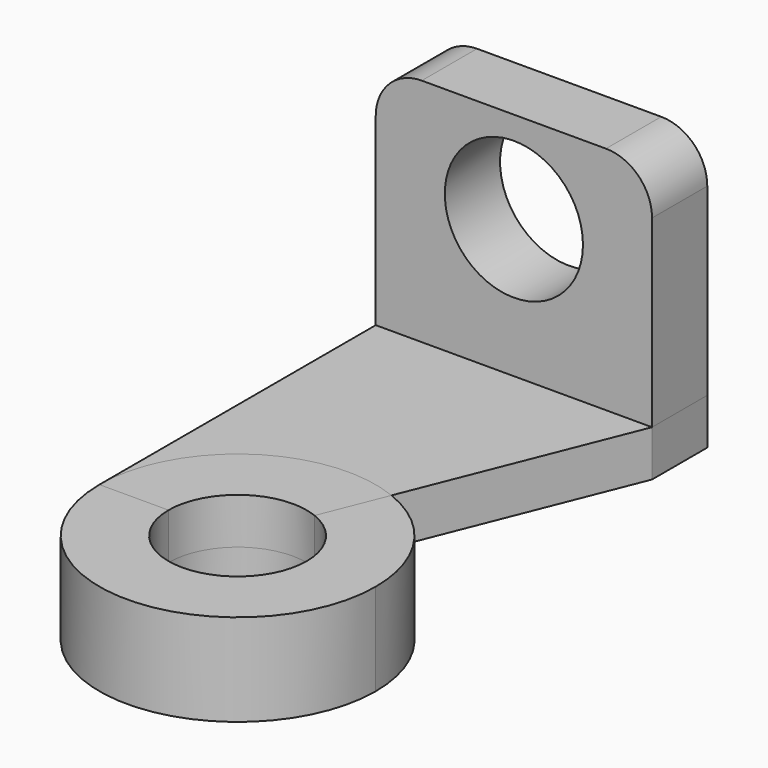
from build123d import *
from build123d import SkipClean  # not in build123d's __all__

# Parameters (mm, degrees)
F1_DEPTH      = 15
F2_R          = 15
F3_DEPTH      = 25
F3_DEPTH_BACK = 25
F6_DEPTH      = 10
F7_DEPTH      = 15
F9_DEPTH      = 10
F10_DEPTH     = 20
F11_DEPTH     = 20


with BuildPart() as f1:
    # F0 (on Front) → F1 (new body)
    with BuildSketch(Plane.XZ):
        with BuildLine():
            ThreePointArc((30, 15), (27.0710678119, 22.0710678119), (20, 25))
            Line((20, 25), (-20, 25))
            ThreePointArc((-20, 25), (-27.0710678119, 22.0710678119), (-30, 15))
            Line((-30, 15), (-30, -25))
            Line((-30, -25), (30, -25))
            Line((30, -25), (30, 15))
        make_face()
    extrude(amount=F1_DEPTH)


with BuildPart() as f3:
    # F2 (on face) → F3 (new body, two sides)
    with BuildSketch(Plane.XZ.offset(15)) as f3_sk:
        with Locations((0, 5)):
            Circle(F2_R)
    extrude(amount=-F3_DEPTH)
    extrude(f3_sk.sketch, amount=F3_DEPTH_BACK)


with BuildPart() as f1_1:
    add(f1.part, clean=False)

    # F4: cut F3
    add(f3.part, mode=Mode.SUBTRACT)



with BuildPart() as f6:
    # F5 (on face) → F6 (new body)
    with BuildSketch(Plane(origin=(0, 0, -25), x_dir=(1, 0, 0), z_dir=(0, 0, -1))):
        Polygon((-30, 90), (-30, 15), (30, 15), (0, 90), align=None)
    extrude(amount=F6_DEPTH)


with BuildPart() as f7:
    # F7 (new): a face of the model
    f7_faces = [f6.part.faces().sort_by_distance(p)[0] for p in [
        (0, -15, -30),
    ]]
    extrude(f7_faces, amount=F7_DEPTH)


with BuildPart() as f6_1:
    add(f6.part, clean=False)

    # F8 (on face) → F9 (cut)
    with BuildSketch(Plane.XY.offset(-25)):
        with BuildLine():
            ThreePointArc((5.5708601453, -76.0728496367), (-8.4094321396, -77.578991543), (-15, -90))
            Line((-15, -90), (0, -90))
            Line((0, -90), (5.5708601453, -76.0728496367))
        make_face()
    extrude(amount=-F9_DEPTH, mode=Mode.SUBTRACT)


with BuildPart() as f1_2:
    add(f1_1.part, clean=False)

    with SkipClean():  # cleaning this boolean's faces spoils the solid; the shape is the same uncleaned
        add(f6_1.part)  # F10 merges F6

    with SkipClean():  # cleaning this boolean's faces spoils the solid; the shape is the same uncleaned
        add(f7.part)  # F10 merges F7
    # F8 (on face) → F10 (join)
    with BuildSketch(Plane.XY.offset(-25)):
        with BuildLine():
            Line((-15, -90), (-30, -90))
            ThreePointArc((-30, -90), (0, -120), (30, -90))
            ThreePointArc((30, -90), (24.8420169141, -73.1811357208), (11.1417202906, -62.1456992734))
            Line((11.1417202906, -62.1456992734), (5.5708601453, -76.0728496367))
            ThreePointArc((5.5708601453, -76.0728496367), (12.421008457, -81.5905678604), (15, -90))
            ThreePointArc((15, -90), (0, -105), (-15, -90))
        make_face()
    with SkipClean():  # cleaning this boolean's faces spoils the solid; the shape is the same uncleaned
        extrude(amount=-F10_DEPTH)

    # F8 (on face) → F11 (join)
    with BuildSketch(Plane.XY.offset(-25)):
        with BuildLine():
            ThreePointArc((11.1417202906, -62.1456992734), (-16.8188642792, -65.1579830859), (-30, -90))
            Line((-30, -90), (-15, -90))
            ThreePointArc((-15, -90), (-8.4094321396, -77.578991543), (5.5708601453, -76.0728496367))
            Line((5.5708601453, -76.0728496367), (11.1417202906, -62.1456992734))
        make_face()
    with SkipClean():  # cleaning this boolean's faces spoils the solid; the shape is the same uncleaned
        extrude(amount=-F11_DEPTH)


solid = f1_2.part
